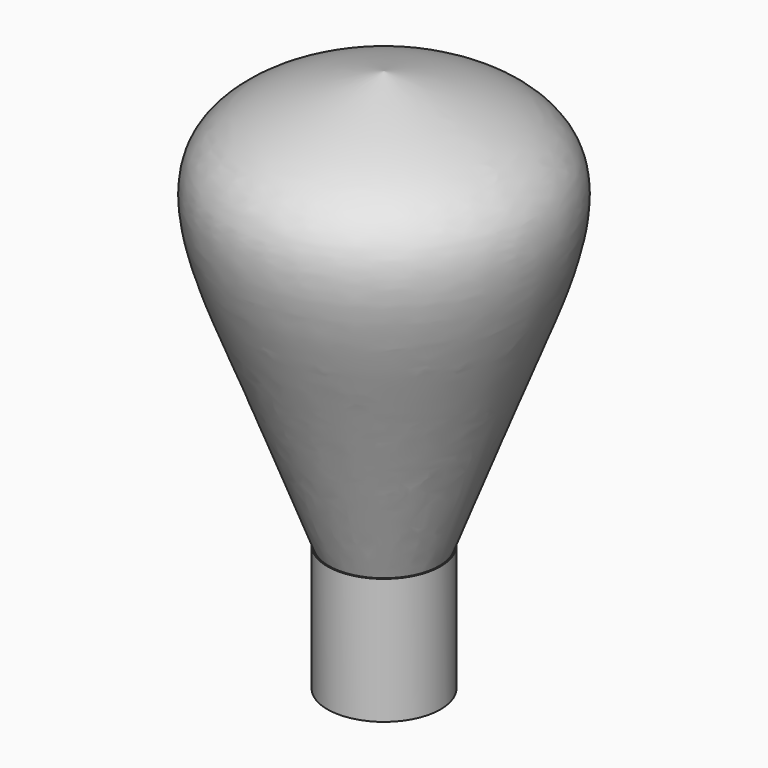
from build123d import *

# Parameters (mm, degrees)
F0_R     = 13.5
F1_DEPTH = 30


# Not quite as in the source:
# - a feature of the source that left no trace in its solid (it failed there, or was rolled back) is left out


with BuildPart() as f1:
    # F0 (on Top) → F1 (new body)
    with BuildSketch(Plane.XY):
        Circle(F0_R)
    extrude(amount=F1_DEPTH)

    # F2 (on Front) → F3 (revolve)
    with BuildSketch(Plane.XZ):
        with BuildLine():
            Line((0, 129.5523982495), (0, 29.5523982495))
            Line((0, 29.5523982495), (13.0988145247, 29.8015400767))
            add(Edge.make_bspline(
                [(13.0988145247, 29.8015400767), (18.3718086188, 43.6941485489), (28.5364277681, 70.4745832678), (47.5999218103, 117.6780805375), (15.9351718164, 125.5771964898), (0, 129.5523982495)],
                knots=[0, 0, 0, 0, 0.3487388383, 0.6722551572, 1, 1, 1, 1], degree=3))
        make_face()
    revolve(axis=Axis((0, 0, 79.5523982495), (0, 0, 1)))


solid = f1.part
